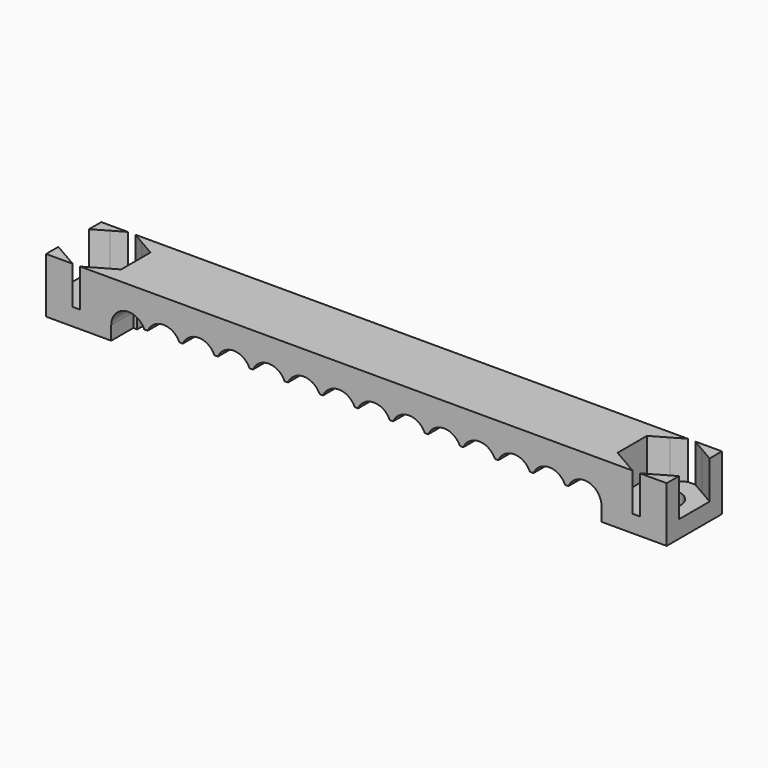
from build123d import *

# Parameters (mm, degrees)
F1_DEPTH = 5
F3_DEPTH = 2
F5_DEPTH = 2.75
F6_R     = 1.2
F7_DEPTH = 5
F8_DEPTH = 1


with BuildPart() as f1:
    # F0 (on Front) → F1 (new body)
    with BuildSketch(Plane.XZ):
        with BuildLine():
            ThreePointArc((-2.24, 1.27), (-1.27, 2.24), (-0.3, 1.27))
            Line((-0.3, 1.27), (0.3, 1.27))
            ThreePointArc((0.3, 1.27), (1.27, 2.24), (2.24, 1.27))
            Line((2.24, 1.27), (2.84, 1.27))
            ThreePointArc((2.84, 1.27), (3.81, 2.24), (4.78, 1.27))
            Line((4.78, 1.27), (5.38, 1.27))
            ThreePointArc((5.38, 1.27), (6.35, 2.24), (7.32, 1.27))
            Line((7.32, 1.27), (7.92, 1.27))
            ThreePointArc((7.92, 1.27), (8.89, 2.24), (9.86, 1.27))
            Line((9.86, 1.27), (10.46, 1.27))
            ThreePointArc((10.46, 1.27), (11.43, 2.24), (12.4, 1.27))
            Line((12.4, 1.27), (13, 1.27))
            ThreePointArc((13, 1.27), (13.97, 2.24), (14.94, 1.27))
            Line((14.94, 1.27), (15.54, 1.27))
            ThreePointArc((15.54, 1.27), (16.51, 2.24), (17.48, 1.27))
            Line((17.48, 1.27), (22.48, 1.27))
            Line((22.48, 1.27), (22.48, 4.27))
            Line((22.48, 4.27), (-22.48, 4.27))
            Line((-22.48, 4.27), (-22.48, 1.27))
            Line((-22.48, 1.27), (-17.48, 1.27))
            ThreePointArc((-17.48, 1.27), (-16.51, 2.24), (-15.54, 1.27))
            Line((-15.54, 1.27), (-14.94, 1.27))
            ThreePointArc((-14.94, 1.27), (-13.97, 2.24), (-13, 1.27))
            Line((-13, 1.27), (-12.4, 1.27))
            ThreePointArc((-12.4, 1.27), (-11.43, 2.24), (-10.46, 1.27))
            Line((-10.46, 1.27), (-9.86, 1.27))
            ThreePointArc((-9.86, 1.27), (-8.89, 2.24), (-7.92, 1.27))
            Line((-7.92, 1.27), (-7.32, 1.27))
            ThreePointArc((-7.32, 1.27), (-6.35, 2.24), (-5.38, 1.27))
            Line((-5.38, 1.27), (-4.78, 1.27))
            ThreePointArc((-4.78, 1.27), (-3.81, 2.24), (-2.84, 1.27))
            Line((-2.84, 1.27), (-2.24, 1.27))
        make_face()
    extrude(amount=F1_DEPTH)

    # F2 (on face) → F3 (cut)
    with BuildSketch(Plane.XZ.offset(5)):
        with BuildLine():
            Line((-16.51, 1.27), (-15.26, 1.27))
            ThreePointArc((-15.26, 1.27), (-15.2863671088, 1.5253870546), (-15.3643560763, 1.77))
            Line((-15.3643560763, 1.77), (-16.51, 1.77))
            Line((-16.51, 1.77), (-16.51, 1.27))
        make_face()
        with BuildLine():
            ThreePointArc((-15.3643560763, 1.77), (-17.7336328912, 1.0146129454), (-15.26, 1.27))
            Line((-15.26, 1.27), (-16.51, 1.27))
            Line((-16.51, 1.27), (-16.51, 1.77))
            Line((-16.51, 1.77), (-15.3643560763, 1.77))
        make_face()
        with BuildLine():
            ThreePointArc((-15.3643560763, 1.77), (-15.2863671088, 1.5253870546), (-15.26, 1.27))
            Line((-15.26, 1.27), (-15.22, 1.27))
            ThreePointArc((-15.22, 1.27), (-15.1936328912, 1.5253870546), (-15.1156439237, 1.77))
            Line((-15.1156439237, 1.77), (-15.3643560763, 1.77))
        make_face()
        with BuildLine():
            Line((-12.72, 1.27), (-15.22, 1.27))
            ThreePointArc((-15.22, 1.27), (-13.97, 0.02), (-12.72, 1.27))
        make_face()
        with BuildLine():
            ThreePointArc((-15.1156439237, 1.77), (-15.1936328912, 1.5253870546), (-15.22, 1.27))
            Line((-15.22, 1.27), (-12.72, 1.27))
            ThreePointArc((-12.72, 1.27), (-12.7463671088, 1.5253870546), (-12.8243560763, 1.77))
            Line((-12.8243560763, 1.77), (-15.1156439237, 1.77))
        make_face()
        with BuildLine():
            ThreePointArc((-12.8243560763, 1.77), (-13.97, 2.52), (-15.1156439237, 1.77))
            Line((-15.1156439237, 1.77), (-12.8243560763, 1.77))
        make_face()
        with BuildLine():
            ThreePointArc((-12.8243560763, 1.77), (-12.7463671088, 1.5253870546), (-12.72, 1.27))
            Line((-12.72, 1.27), (-12.68, 1.27))
            ThreePointArc((-12.68, 1.27), (-12.6536328912, 1.5253870546), (-12.5756439237, 1.77))
            Line((-12.5756439237, 1.77), (-12.8243560763, 1.77))
        make_face()
        with BuildLine():
            Line((-10.18, 1.27), (-12.68, 1.27))
            ThreePointArc((-12.68, 1.27), (-11.43, 0.02), (-10.18, 1.27))
        make_face()
        with BuildLine():
            ThreePointArc((-12.5756439237, 1.77), (-12.6536328912, 1.5253870546), (-12.68, 1.27))
            Line((-12.68, 1.27), (-10.18, 1.27))
            ThreePointArc((-10.18, 1.27), (-10.2063671088, 1.5253870546), (-10.2843560763, 1.77))
            Line((-10.2843560763, 1.77), (-12.5756439237, 1.77))
        make_face()
        with BuildLine():
            ThreePointArc((-10.2843560763, 1.77), (-11.43, 2.52), (-12.5756439237, 1.77))
            Line((-12.5756439237, 1.77), (-10.2843560763, 1.77))
        make_face()
        with BuildLine():
            ThreePointArc((-10.2843560763, 1.77), (-10.2063671088, 1.5253870546), (-10.18, 1.27))
            Line((-10.18, 1.27), (-10.14, 1.27))
            ThreePointArc((-10.14, 1.27), (-10.1136328912, 1.5253870546), (-10.0356439237, 1.77))
            Line((-10.0356439237, 1.77), (-10.2843560763, 1.77))
        make_face()
        with BuildLine():
            Line((-7.64, 1.27), (-10.14, 1.27))
            ThreePointArc((-10.14, 1.27), (-8.89, 0.02), (-7.64, 1.27))
        make_face()
        with BuildLine():
            ThreePointArc((-10.0356439237, 1.77), (-10.1136328912, 1.5253870546), (-10.14, 1.27))
            Line((-10.14, 1.27), (-7.64, 1.27))
            ThreePointArc((-7.64, 1.27), (-7.6663671088, 1.5253870546), (-7.7443560763, 1.77))
            Line((-7.7443560763, 1.77), (-10.0356439237, 1.77))
        make_face()
        with BuildLine():
            ThreePointArc((-7.7443560763, 1.77), (-8.89, 2.52), (-10.0356439237, 1.77))
            Line((-10.0356439237, 1.77), (-7.7443560763, 1.77))
        make_face()
        with BuildLine():
            ThreePointArc((-7.7443560763, 1.77), (-7.6663671088, 1.5253870546), (-7.64, 1.27))
            Line((-7.64, 1.27), (-7.6, 1.27))
            ThreePointArc((-7.6, 1.27), (-7.5736328912, 1.5253870546), (-7.4956439237, 1.77))
            Line((-7.4956439237, 1.77), (-7.7443560763, 1.77))
        make_face()
        with BuildLine():
            Line((-5.1, 1.27), (-7.6, 1.27))
            ThreePointArc((-7.6, 1.27), (-6.35, 0.02), (-5.1, 1.27))
        make_face()
        with BuildLine():
            ThreePointArc((-7.4956439237, 1.77), (-7.5736328912, 1.5253870546), (-7.6, 1.27))
            Line((-7.6, 1.27), (-5.1, 1.27))
            ThreePointArc((-5.1, 1.27), (-5.1263671088, 1.5253870546), (-5.2043560763, 1.77))
            Line((-5.2043560763, 1.77), (-7.4956439237, 1.77))
        make_face()
        with BuildLine():
            ThreePointArc((-5.2043560763, 1.77), (-6.35, 2.52), (-7.4956439237, 1.77))
            Line((-7.4956439237, 1.77), (-5.2043560763, 1.77))
        make_face()
        with BuildLine():
            ThreePointArc((-5.2043560763, 1.77), (-5.1263671088, 1.5253870546), (-5.1, 1.27))
            Line((-5.1, 1.27), (-5.06, 1.27))
            ThreePointArc((-5.06, 1.27), (-5.0336328912, 1.5253870546), (-4.9556439237, 1.77))
            Line((-4.9556439237, 1.77), (-5.2043560763, 1.77))
        make_face()
        with BuildLine():
            Line((-2.56, 1.27), (-5.06, 1.27))
            ThreePointArc((-5.06, 1.27), (-3.81, 0.02), (-2.56, 1.27))
        make_face()
        with BuildLine():
            ThreePointArc((-4.9556439237, 1.77), (-5.0336328912, 1.5253870546), (-5.06, 1.27))
            Line((-5.06, 1.27), (-2.56, 1.27))
            ThreePointArc((-2.56, 1.27), (-2.5863671088, 1.5253870546), (-2.6643560763, 1.77))
            Line((-2.6643560763, 1.77), (-4.9556439237, 1.77))
        make_face()
        with BuildLine():
            ThreePointArc((-2.6643560763, 1.77), (-3.81, 2.52), (-4.9556439237, 1.77))
            Line((-4.9556439237, 1.77), (-2.6643560763, 1.77))
        make_face()
        with BuildLine():
            ThreePointArc((-2.6643560763, 1.77), (-2.5863671088, 1.5253870546), (-2.56, 1.27))
            Line((-2.56, 1.27), (-2.52, 1.27))
            ThreePointArc((-2.52, 1.27), (-2.4936328912, 1.5253870546), (-2.4156439237, 1.77))
            Line((-2.4156439237, 1.77), (-2.6643560763, 1.77))
        make_face()
        with BuildLine():
            Line((-0.02, 1.27), (-2.52, 1.27))
            ThreePointArc((-2.52, 1.27), (-1.27, 0.02), (-0.02, 1.27))
        make_face()
        with BuildLine():
            ThreePointArc((-2.4156439237, 1.77), (-2.4936328912, 1.5253870546), (-2.52, 1.27))
            Line((-2.52, 1.27), (-0.02, 1.27))
            ThreePointArc((-0.02, 1.27), (-0.0463671088, 1.5253870546), (-0.1243560763, 1.77))
            Line((-0.1243560763, 1.77), (-2.4156439237, 1.77))
        make_face()
        with BuildLine():
            ThreePointArc((-0.1243560763, 1.77), (-1.27, 2.52), (-2.4156439237, 1.77))
            Line((-2.4156439237, 1.77), (-0.1243560763, 1.77))
        make_face()
        with BuildLine():
            ThreePointArc((-0.1243560763, 1.77), (-0.0463671088, 1.5253870546), (-0.02, 1.27))
            Line((-0.02, 1.27), (0.02, 1.27))
            ThreePointArc((0.02, 1.27), (0.0463671088, 1.5253870546), (0.1243560763, 1.77))
            Line((0.1243560763, 1.77), (-0.1243560763, 1.77))
        make_face()
        with BuildLine():
            Line((2.52, 1.27), (0.02, 1.27))
            ThreePointArc((0.02, 1.27), (1.27, 0.02), (2.52, 1.27))
        make_face()
        with BuildLine():
            ThreePointArc((0.1243560763, 1.77), (0.0463671088, 1.5253870546), (0.02, 1.27))
            Line((0.02, 1.27), (2.52, 1.27))
            ThreePointArc((2.52, 1.27), (2.4936328912, 1.5253870546), (2.4156439237, 1.77))
            Line((2.4156439237, 1.77), (0.1243560763, 1.77))
        make_face()
        with BuildLine():
            ThreePointArc((2.4156439237, 1.77), (1.27, 2.52), (0.1243560763, 1.77))
            Line((0.1243560763, 1.77), (2.4156439237, 1.77))
        make_face()
        with BuildLine():
            ThreePointArc((2.4156439237, 1.77), (2.4936328912, 1.5253870546), (2.52, 1.27))
            Line((2.52, 1.27), (2.56, 1.27))
            ThreePointArc((2.56, 1.27), (2.5863671088, 1.5253870546), (2.6643560763, 1.77))
            Line((2.6643560763, 1.77), (2.4156439237, 1.77))
        make_face()
        with BuildLine():
            Line((5.06, 1.27), (2.56, 1.27))
            ThreePointArc((2.56, 1.27), (3.81, 0.02), (5.06, 1.27))
        make_face()
        with BuildLine():
            ThreePointArc((2.6643560763, 1.77), (2.5863671088, 1.5253870546), (2.56, 1.27))
            Line((2.56, 1.27), (5.06, 1.27))
            ThreePointArc((5.06, 1.27), (5.0336328912, 1.5253870546), (4.9556439237, 1.77))
            Line((4.9556439237, 1.77), (2.6643560763, 1.77))
        make_face()
        with BuildLine():
            ThreePointArc((4.9556439237, 1.77), (3.81, 2.52), (2.6643560763, 1.77))
            Line((2.6643560763, 1.77), (4.9556439237, 1.77))
        make_face()
        with BuildLine():
            ThreePointArc((4.9556439237, 1.77), (5.0336328912, 1.5253870546), (5.06, 1.27))
            Line((5.06, 1.27), (5.1, 1.27))
            ThreePointArc((5.1, 1.27), (5.1263671088, 1.5253870546), (5.2043560763, 1.77))
            Line((5.2043560763, 1.77), (4.9556439237, 1.77))
        make_face()
        with BuildLine():
            Line((7.6, 1.27), (5.1, 1.27))
            ThreePointArc((5.1, 1.27), (6.35, 0.02), (7.6, 1.27))
        make_face()
        with BuildLine():
            ThreePointArc((5.2043560763, 1.77), (5.1263671088, 1.5253870546), (5.1, 1.27))
            Line((5.1, 1.27), (7.6, 1.27))
            ThreePointArc((7.6, 1.27), (7.5736328912, 1.5253870546), (7.4956439237, 1.77))
            Line((7.4956439237, 1.77), (5.2043560763, 1.77))
        make_face()
        with BuildLine():
            ThreePointArc((7.4956439237, 1.77), (6.35, 2.52), (5.2043560763, 1.77))
            Line((5.2043560763, 1.77), (7.4956439237, 1.77))
        make_face()
        with BuildLine():
            ThreePointArc((7.4956439237, 1.77), (7.5736328912, 1.5253870546), (7.6, 1.27))
            Line((7.6, 1.27), (7.64, 1.27))
            ThreePointArc((7.64, 1.27), (7.6663671088, 1.5253870546), (7.7443560763, 1.77))
            Line((7.7443560763, 1.77), (7.4956439237, 1.77))
        make_face()
        with BuildLine():
            Line((10.14, 1.27), (7.64, 1.27))
            ThreePointArc((7.64, 1.27), (8.89, 0.02), (10.14, 1.27))
        make_face()
        with BuildLine():
            ThreePointArc((7.7443560763, 1.77), (7.6663671088, 1.5253870546), (7.64, 1.27))
            Line((7.64, 1.27), (10.14, 1.27))
            ThreePointArc((10.14, 1.27), (10.1136328912, 1.5253870546), (10.0356439237, 1.77))
            Line((10.0356439237, 1.77), (7.7443560763, 1.77))
        make_face()
        with BuildLine():
            ThreePointArc((10.0356439237, 1.77), (8.89, 2.52), (7.7443560763, 1.77))
            Line((7.7443560763, 1.77), (10.0356439237, 1.77))
        make_face()
        with BuildLine():
            ThreePointArc((10.0356439237, 1.77), (10.1136328912, 1.5253870546), (10.14, 1.27))
            Line((10.14, 1.27), (10.18, 1.27))
            ThreePointArc((10.18, 1.27), (10.2063671088, 1.5253870546), (10.2843560763, 1.77))
            Line((10.2843560763, 1.77), (10.0356439237, 1.77))
        make_face()
        with BuildLine():
            Line((12.68, 1.27), (10.18, 1.27))
            ThreePointArc((10.18, 1.27), (11.43, 0.02), (12.68, 1.27))
        make_face()
        with BuildLine():
            ThreePointArc((10.2843560763, 1.77), (10.2063671088, 1.5253870546), (10.18, 1.27))
            Line((10.18, 1.27), (12.68, 1.27))
            ThreePointArc((12.68, 1.27), (12.6536328912, 1.5253870546), (12.5756439237, 1.77))
            Line((12.5756439237, 1.77), (10.2843560763, 1.77))
        make_face()
        with BuildLine():
            ThreePointArc((12.5756439237, 1.77), (11.43, 2.52), (10.2843560763, 1.77))
            Line((10.2843560763, 1.77), (12.5756439237, 1.77))
        make_face()
        with BuildLine():
            ThreePointArc((12.5756439237, 1.77), (12.6536328912, 1.5253870546), (12.68, 1.27))
            Line((12.68, 1.27), (12.72, 1.27))
            ThreePointArc((12.72, 1.27), (12.7463671088, 1.5253870546), (12.8243560763, 1.77))
            Line((12.8243560763, 1.77), (12.5756439237, 1.77))
        make_face()
        with BuildLine():
            Line((15.22, 1.27), (12.72, 1.27))
            ThreePointArc((12.72, 1.27), (13.97, 0.02), (15.22, 1.27))
        make_face()
        with BuildLine():
            ThreePointArc((12.8243560763, 1.77), (12.7463671088, 1.5253870546), (12.72, 1.27))
            Line((12.72, 1.27), (15.22, 1.27))
            ThreePointArc((15.22, 1.27), (15.1936328912, 1.5253870546), (15.1156439237, 1.77))
            Line((15.1156439237, 1.77), (12.8243560763, 1.77))
        make_face()
        with BuildLine():
            ThreePointArc((15.1156439237, 1.77), (13.97, 2.52), (12.8243560763, 1.77))
            Line((12.8243560763, 1.77), (15.1156439237, 1.77))
        make_face()
        with BuildLine():
            ThreePointArc((15.1156439237, 1.77), (15.1936328912, 1.5253870546), (15.22, 1.27))
            Line((15.22, 1.27), (15.26, 1.27))
            ThreePointArc((15.26, 1.27), (15.2863671088, 1.5253870546), (15.3643560763, 1.77))
            Line((15.3643560763, 1.77), (15.1156439237, 1.77))
        make_face()
        with BuildLine():
            Line((16.51, 1.27), (15.26, 1.27))
            ThreePointArc((15.26, 1.27), (16.51, 0.02), (17.76, 1.27))
            ThreePointArc((17.76, 1.27), (16.7653870546, 2.4936328912), (15.3643560763, 1.77))
            Line((15.3643560763, 1.77), (16.51, 1.77))
            Line((16.51, 1.77), (16.51, 1.27))
        make_face()
        with BuildLine():
            ThreePointArc((15.3643560763, 1.77), (15.2863671088, 1.5253870546), (15.26, 1.27))
            Line((15.26, 1.27), (16.51, 1.27))
            Line((16.51, 1.27), (16.51, 1.77))
            Line((16.51, 1.77), (15.3643560763, 1.77))
        make_face()
    extrude(amount=-F3_DEPTH, mode=Mode.SUBTRACT)

    # F4 (on face) → F5 (cut)
    with BuildSketch(Plane.XY.offset(4.27)):
        with BuildLine():
            ThreePointArc((21.4299999725, -4.4918584446), (22.2718584208, -3.6500000137), (22.58, -2.5))
            ThreePointArc((22.58, -2.5), (22.271858109, -1.3499994462), (21.4299988924, -0.5081409318))
            ThreePointArc((21.4299988924, -0.5081409318), (20.280000147, -0.2), (19.1300013622, -0.5081407848))
            ThreePointArc((19.1300013622, -0.5081407848), (18.2881419645, -1.3499993189), (17.98, -2.5))
            ThreePointArc((17.98, -2.5), (18.2881415897, -3.6500000318), (19.1300000637, -4.4918584655))
            ThreePointArc((19.1300000637, -4.4918584655), (20.2800000209, -4.8), (21.4299999725, -4.4918584446))
        make_face()
        with BuildLine():
            Line((22.58, -3.8279056191), (22.58, -2.5))
            ThreePointArc((22.58, -2.5), (22.2718584208, -3.6500000137), (21.4299999725, -4.4918584446))
            Line((21.4299999725, -4.4918584446), (22.58, -3.8279056191))
        make_face()
        with BuildLine():
            ThreePointArc((21.4299988924, -0.5081409318), (22.271858109, -1.3499994462), (22.58, -2.5))
            Line((22.58, -2.5), (22.58, -1.1720943809))
            Line((22.58, -1.1720943809), (21.4299988924, -0.5081409318))
        make_face()
        with BuildLine():
            ThreePointArc((19.1300013622, -0.5081407848), (20.280000147, -0.2), (21.4299988924, -0.5081409318))
            Line((21.4299988924, -0.5081409318), (20.28, 0.1558112383))
            Line((20.28, 0.1558112383), (19.1300013622, -0.5081407848))
        make_face()
        with BuildLine():
            Line((20.28, -5.1558112383), (21.4299999725, -4.4918584446))
            ThreePointArc((21.4299999725, -4.4918584446), (20.2800000209, -4.8), (19.1300000637, -4.4918584655))
            Line((19.1300000637, -4.4918584655), (20.28, -5.1558112383))
        make_face()
        with BuildLine():
            ThreePointArc((17.98, -2.5), (18.2881419645, -1.3499993189), (19.1300013622, -0.5081407848))
            Line((19.1300013622, -0.5081407848), (17.98, -1.1720943809))
            Line((17.98, -1.1720943809), (17.98, -2.5))
        make_face()
        with BuildLine():
            Line((17.98, -3.8279056191), (19.1300000637, -4.4918584655))
            ThreePointArc((19.1300000637, -4.4918584655), (18.2881415897, -3.6500000318), (17.98, -2.5))
            Line((17.98, -2.5), (17.98, -3.8279056191))
        make_face()
        with BuildLine():
            ThreePointArc((-19.1300000861, -4.4918584784), (-18.2881415961, -3.650000043), (-17.98, -2.5))
            ThreePointArc((-17.98, -2.5), (-18.2881415051, -1.3500001146), (-19.1299997708, -0.5081417036))
            ThreePointArc((-19.1299997708, -0.5081417036), (-20.2799996458, -0.2), (-21.4299996157, -0.5081413494))
            ThreePointArc((-21.4299996157, -0.5081413494), (-22.2718583178, -1.3499998079), (-22.58, -2.5))
            ThreePointArc((-22.58, -2.5), (-22.2718584103, -3.6500000318), (-21.4299999363, -4.4918584655))
            ThreePointArc((-21.4299999363, -4.4918584655), (-20.2800000129, -4.8), (-19.1300000861, -4.4918584784))
        make_face()
        with BuildLine():
            Line((-17.98, -3.8279056191), (-17.98, -2.5))
            ThreePointArc((-17.98, -2.5), (-18.2881415961, -3.650000043), (-19.1300000861, -4.4918584784))
            Line((-19.1300000861, -4.4918584784), (-17.98, -3.8279056191))
        make_face()
        with BuildLine():
            ThreePointArc((-19.1299997708, -0.5081417036), (-18.2881415051, -1.3500001146), (-17.98, -2.5))
            Line((-17.98, -2.5), (-17.98, -1.1720943809))
            Line((-17.98, -1.1720943809), (-19.1299997708, -0.5081417036))
        make_face()
        with BuildLine():
            ThreePointArc((-21.4299996157, -0.5081413494), (-20.2799996458, -0.2), (-19.1299997708, -0.5081417036))
            Line((-19.1299997708, -0.5081417036), (-20.28, 0.1558112383))
            Line((-20.28, 0.1558112383), (-21.4299996157, -0.5081413494))
        make_face()
        with BuildLine():
            Line((-20.28, -5.1558112383), (-19.1300000861, -4.4918584784))
            ThreePointArc((-19.1300000861, -4.4918584784), (-20.2800000129, -4.8), (-21.4299999363, -4.4918584655))
            Line((-21.4299999363, -4.4918584655), (-20.28, -5.1558112383))
        make_face()
        with BuildLine():
            ThreePointArc((-22.58, -2.5), (-22.2718583178, -1.3499998079), (-21.4299996157, -0.5081413494))
            Line((-21.4299996157, -0.5081413494), (-22.58, -1.1720943809))
            Line((-22.58, -1.1720943809), (-22.58, -2.5))
        make_face()
        with BuildLine():
            Line((-22.58, -3.8279056191), (-21.4299999363, -4.4918584655))
            ThreePointArc((-21.4299999363, -4.4918584655), (-22.2718584103, -3.6500000318), (-22.58, -2.5))
            Line((-22.58, -2.5), (-22.58, -3.8279056191))
        make_face()
    extrude(amount=-F5_DEPTH, mode=Mode.SUBTRACT)

    # F6 (on Top) → F7 (cut)
    with BuildSketch(Plane.XY):
        with Locations((-20.28, -2.5)):
            Circle(F6_R)
        with Locations((20.28, -2.5)):
            Circle(F6_R)
    extrude(amount=F7_DEPTH, mode=Mode.SUBTRACT)

    # F8 (add): faces of the model
    f8_faces = [f1.faces().sort_by_distance(p)[0] for p in [
        (-19.98, -0.0707106781, 1.27),
        (19.98, -0.0707106781, 1.27),
    ]]
    extrude(f8_faces, amount=F8_DEPTH)


solid = f1.part
